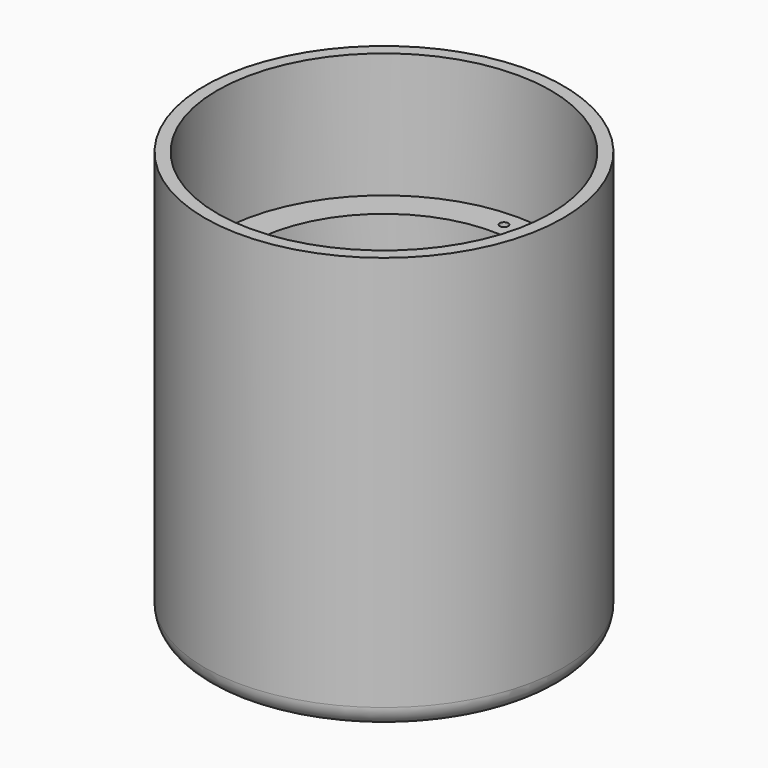
from build123d import *

# Parameters (mm, degrees)
F0_R     = 43
F0_R_2   = 40
F1_DEPTH = 30
F2_DEPTH = 70
F0_R_3   = 1
F0_R_4   = 32.5
F3_DEPTH = 10
F4_R     = 43
F4_R_2   = 40
F4_R_3   = 5
F5_DEPTH = 3
F6_R     = 5


with BuildPart() as f1:
    # F0 (on Top) → F1 (new body)
    with BuildSketch(Plane.XY):
        Circle(F0_R)
        Circle(F0_R_2, mode=Mode.SUBTRACT)
    extrude(amount=F1_DEPTH)

    # F0 (on Top) → F2 (join)
    with BuildSketch(Plane.XY):
        Circle(F0_R)
        Circle(F0_R_2, mode=Mode.SUBTRACT)
    extrude(amount=-F2_DEPTH)

    # F0 (on Top) → F3 (join)
    with BuildSketch(Plane.XY):
        Circle(F0_R_2)
        with Locations((0, -36)):
            Circle(F0_R_3, mode=Mode.SUBTRACT)
        with Locations((-36, 0)):
            Circle(F0_R_3, mode=Mode.SUBTRACT)
        Circle(F0_R_4, mode=Mode.SUBTRACT)
        with Locations((36, 0)):
            Circle(F0_R_3, mode=Mode.SUBTRACT)
        with Locations((0, 36)):
            Circle(F0_R_3, mode=Mode.SUBTRACT)
    extrude(amount=-F3_DEPTH)

    # F4 (on face) → F5 (join)
    with BuildSketch(Plane(origin=(0, 0, -70), x_dir=(1, 0, 0), z_dir=(0, 0, -1))):
        Circle(F4_R)
        Circle(F4_R_2, mode=Mode.SUBTRACT)
        Circle(F4_R_2)
        Circle(F4_R_3, mode=Mode.SUBTRACT)
    extrude(amount=-F5_DEPTH)

    # F6
    f6_edges = [f1.edges().sort_by_distance(p)[0] for p in [
        (-43, 0, -70),
        (-40, 0, -67),
    ]]
    fillet(f6_edges, radius=F6_R)


solid = f1.part
